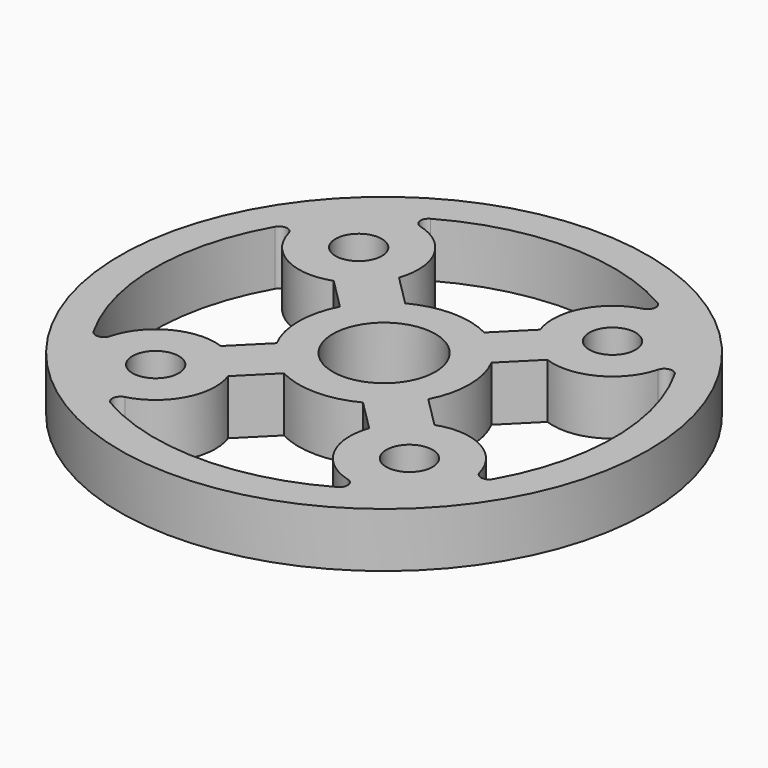
from build123d import *

# Parameters (mm, degrees)
F0_R            = 24.51608
F0_R_2          = 2.15265
F0_R_3          = 4.7625
F1_DEPTH        = 5.08
F3_DEPTH        = 5.08
F3_COPIES_COUNT = 4
F4_R            = 0.762


# Not quite as in the source:
# - a pattern or mirror of a feature is missing from the dataset's text; its kind, count and spacing are read off the source's solid


with BuildPart() as f1:
    # F0 (on Top) → F1 (new body)
    with BuildSketch(Plane.XY):
        Circle(F0_R)
        with Locations((-11.7865906, -11.7865906)):
            Circle(F0_R_2, mode=Mode.SUBTRACT)
        with Locations((11.7865906, -11.7865906)):
            Circle(F0_R_2, mode=Mode.SUBTRACT)
        with Locations((-11.7865906, 11.7865906)):
            Circle(F0_R_2, mode=Mode.SUBTRACT)
        Circle(F0_R_3, mode=Mode.SUBTRACT)
        with Locations((11.7865906, 11.7865906)):
            Circle(F0_R_2, mode=Mode.SUBTRACT)
    extrude(amount=F1_DEPTH)

    # F2 (on face) → F3 (cut, through all)
    with BuildSketch(Plane.XY.offset(5.08)):
        with BuildLine():
            ThreePointArc((-12.5005198818, 17.2967828873), (-7.4612395718, 15.2741760893), (-6.553034663, 9.9206307084))
            Line((-6.553034663, 9.9206307084), (-3.6703384477, 7.0379344931))
            ThreePointArc((-3.6703384477, 7.0379344931), (0, 7.9375), (3.6703384477, 7.0379344931))
            Line((3.6703384477, 7.0379344931), (6.553034663, 9.9206307084))
            ThreePointArc((6.553034663, 9.9206307084), (7.4612395718, 15.2741760893), (12.5005198818, 17.2967828873))
            ThreePointArc((12.5005198818, 17.2967828873), (0, 21.34108), (-12.5005198818, 17.2967828873))
        make_face()
    f3 = extrude(amount=-F3_DEPTH, mode=Mode.SUBTRACT)

    # F3_copies: F3 ×4 about axis
    f3_copies_axis = Axis((0, 0, 0), (0, 0, 1))
    for i in range(1, F3_COPIES_COUNT):
        add(f3.rotate(f3_copies_axis, i * 360 / F3_COPIES_COUNT), mode=Mode.SUBTRACT)

    # F4
    f4_edges = [f1.edges().sort_by_distance(p)[0] for p in [
        (-12.50052, 17.296783, 2.54),
        (12.50052, 17.296783, 2.54),
        (-17.296783, -12.50052, 2.54),
        (-17.296783, 12.50052, 2.54),
        (12.50052, -17.296783, 2.54),
        (-12.50052, -17.296783, 2.54),
        (17.296783, 12.50052, 2.54),
        (17.296783, -12.50052, 2.54),
    ]]
    fillet(f4_edges, radius=F4_R)


solid = f1.part
